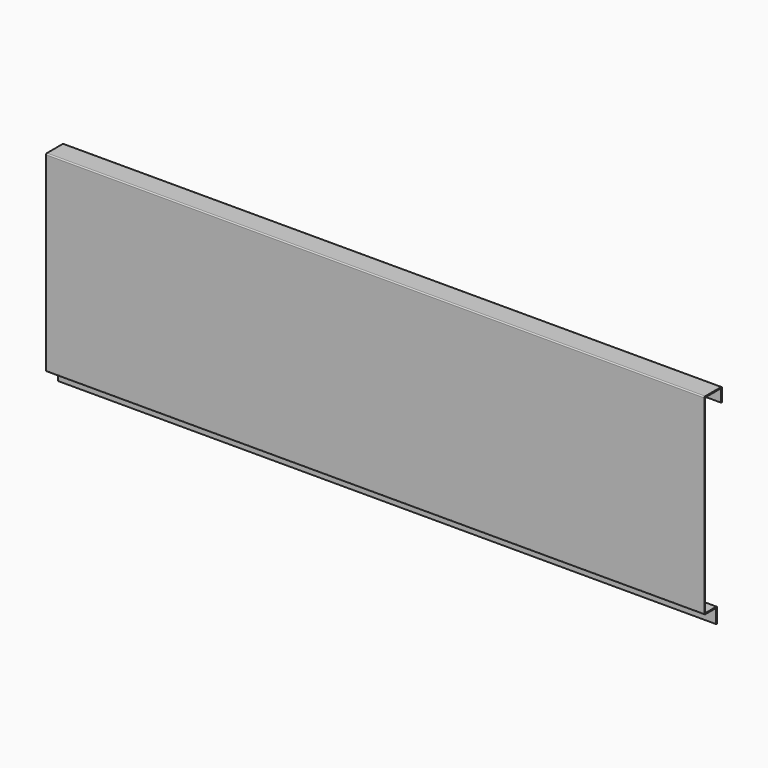
from build123d import *

# Parameters (mm, degrees)
F1_DEPTH = 1200
F3_D     = 8
F4_R     = 2


# Not quite as in the source:
# - a feature names something its author has since deleted; it is built from what else it names


with BuildPart() as f1:
    # F0 (on Right) → F1 (new body)
    with BuildSketch(Plane.YZ):
        Polygon((-18.8378913403, 427.8021101952), (-18.8378913403, 404.8021101952), (-16.8378913403, 404.8021101952), (-16.8378913403, 429.8021101952), (-56.8378913403, 429.8021101952), (-56.8378913403, 79.8021101952), (-29.8378913403, 79.8021101952), (-29.8378913403, 53.8021101952), (-27.8378913403, 53.8021101952), (-27.8378913403, 81.8021101952), (-54.8378913403, 81.8021101952), (-54.8378913403, 427.8021101952), align=None)
    extrude(amount=F1_DEPTH)

    # F3 (through all)
    with Locations(Plane.XZ.offset(29.8378913403)):
        with Locations((433, 66.8021101952), (767, 66.8021101952), (1100, 66.8021101952), (100, 66.8021101952)):
            Hole(F3_D / 2)

    # F4
    f4_edges = [f1.edges().sort_by_distance(p)[0] for p in [
        (600, -56.837891, 429.80211),
        (600, -16.837891, 429.80211),
        (600, -56.837891, 79.80211),
        (600, -27.837891, 81.80211),
        (600, -54.837891, 81.80211),
        (600, -29.837891, 79.80211),
        (600, -18.837891, 427.80211),
        (600, -54.837891, 427.80211),
    ]]
    fillet(f4_edges, radius=F4_R)


solid = f1.part
